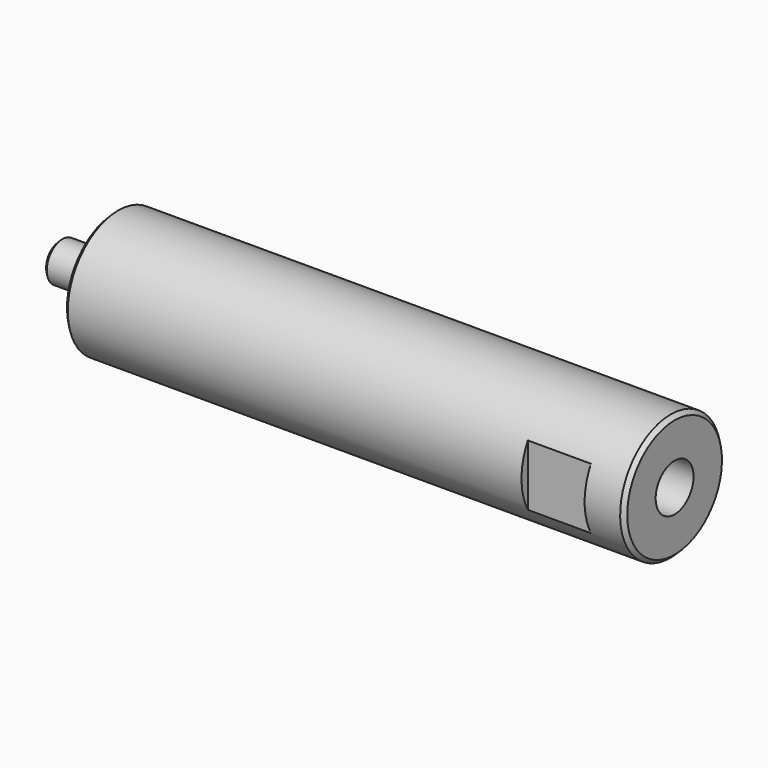
from build123d import *

# Parameters (mm, degrees)
F0_W     = 0.4
F0_H     = 2.066987
F0_W_2   = 6.166988
F0_H_2   = 0.433013
F0_W_3   = 0.433012
F4_DEPTH = 8


with BuildPart() as f1:
    # F0 (on Front) → F1 (revolve)
    with BuildSketch(Plane.XZ):
        Polygon((-25.239477, -88.669804), (-20.739477, -88.669804), (-20.739477, -83.669804), (-90.739477, -83.669804), (-90.739477, -91.669804), (-37.659028, -91.669804), (-36.239477, -89.21107), (-33.239477, -89.21107), (-33.239477, -87.796821), (-25.239477, -87.796821), align=None)
        Polygon((-26.1410899297, -88.669804), (-25.239477, -88.669804), (-25.239477, -87.796821), align=None)
        Polygon((-32.239477, -88.669804), (-26.1410899297, -88.669804), (-25.239477, -87.796821), (-33.239477, -87.796821), (-32.3025853972, -88.7039624297), align=None)
        Polygon((-33.239477, -87.796821), (-33.239477, -89.21107), (-32.3025853972, -88.7039624297), align=None)
        Polygon((-20.739477, -88.669804), (-20.239477, -88.669804), (-20.239477, -84.169804), (-20.739477, -83.669804), align=None)
        Polygon((-90.739477, -91.669804), (-90.739477, -83.669804), (-91.239477, -84.169804), (-91.239477, -87.049804), (-91.239477, -89.169804), (-91.239477, -89.602817), (-91.239477, -91.669804), align=None)
        with Locations((-91.439477, -90.6363105)):
            Rectangle(F0_W, F0_H)
        with BuildLine():
            Line((-91.639477, -89.602817), (-91.239477, -89.602817))
            Line((-91.239477, -89.602817), (-91.239477, -89.169804))
            ThreePointArc((-91.239477, -89.169804), (-91.439477, -89.369804), (-91.639477, -89.169804))
            Line((-91.639477, -89.169804), (-91.639477, -89.602817))
        make_face()
        with Locations((-94.722971, -89.3863105)):
            Rectangle(F0_W_2, F0_H_2)
        with Locations((-94.722971, -90.6363105)):
            Rectangle(F0_W_2, F0_H)
        with Locations((-98.022971, -90.6363105)):
            Rectangle(F0_W_3, F0_H)
        Polygon((-98.239477, -89.602817), (-97.806465, -89.602817), (-97.806465, -89.169804), align=None)
    revolve(axis=Axis((-57.779478, 0, -91.669804), (-1, 0, 0)))

    # F3 (on offset) → F4 (cut)
    with BuildSketch(Plane.YZ.offset(-33.239477)):
        Polygon((-7, -105.1077917218), (-7, -81.2891572714), (-14.8517033085, -81.2891572714), (-15.7914049923, -106.496937573), align=None)
        Polygon((14.2944240943, -81.2891572714), (7, -81.2891572714), (7, -105.1077917218), (14.2944240943, -107.9208105803), align=None)
    extrude(amount=F4_DEPTH, mode=Mode.SUBTRACT)


solid = f1.part
